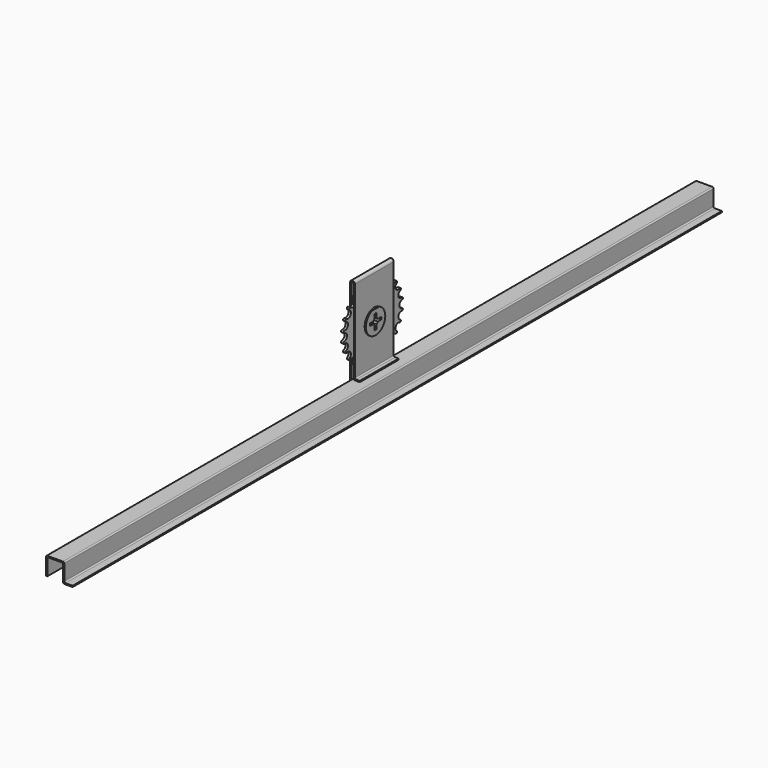
from build123d import *

# Parameters (mm, degrees)
F7_DEPTH      = 335
F1_R          = 1
F3_DEPTH      = 2
F9_DEPTH      = 2
F9_DEPTH_BACK = 4
F10_DEPTH     = 20
F11_DEPTH     = 25
F6_R          = 1


with BuildPart() as f7:
    # F0 (on Front) → F7 (new body, symmetric)
    with BuildSketch(Plane.XZ):
        Polygon((1, 0), (0, 0), (0, -1), (0, -15), (1, -15), (1, -1), (14, -1), (14, -15), (14, -16), (15, -16), (21.9038559089, -16), (21.9038559089, -15), (15, -15), (15, -1), (15, 0), (14, 0), align=None)
    extrude(amount=F7_DEPTH, both=True)

    # F1
    f1_edges = [f7.edges().sort_by_distance(p)[0] for p in [
        (15, 0, 0),
        (0, 0, 0),
        (15, 0, -15),
        (14, 0, -16),
        (14, 0, -1),
    ]]
    fillet(f1_edges, radius=F1_R)


with BuildPart() as f3:
    # F2 (on Right) → F3 (new body)
    with BuildSketch(Plane.YZ):
        with BuildLine():
            ThreePointArc((-29.8037906123, 37.9935767697), (-27, 35), (-29.8037906123, 32.0064232303))
            ThreePointArc((-29.8037906123, 32.0064232303), (-30.6596270407, 30.963583525), (-29.5630457547, 30.1777844881))
            ThreePointArc((-29.5630457547, 30.1777844881), (-26.0799973098, 28.0118857822), (-28.0134563928, 24.3946382584))
            ThreePointArc((-28.0134563928, 24.3946382584), (-28.5702241253, 23.1658256873), (-27.3076281842, 22.6906182246))
            ThreePointArc((-27.3076281842, 22.6906182246), (-23.3826859022, 21.5), (-24.3140514145, 17.5055911631))
            ThreePointArc((-24.3140514145, 17.5055911631), (-24.5338076503, 16.1745472721), (-23.1912408809, 16.0423159868))
            ThreePointArc((-23.1912408809, 16.0423159868), (-19.091883092, 15.908116908), (-18.9576840132, 11.8087591191))
            ThreePointArc((-18.9576840132, 11.8087591191), (-18.8254527279, 10.4661923497), (-17.4944088369, 10.6859485855))
            ThreePointArc((-17.4944088369, 10.6859485855), (-13.5, 11.6173140978), (-12.3093817754, 7.6923718158))
            ThreePointArc((-12.3093817754, 7.6923718158), (-11.8341743127, 6.4297758747), (-10.6053617416, 6.9865436072))
            ThreePointArc((-10.6053617416, 6.9865436072), (-6.9881142178, 8.9200026902), (-4.8222155119, 5.4369542453))
            ThreePointArc((-4.8222155119, 5.4369542453), (-4.036416475, 4.3403729593), (-2.9935767697, 5.1962093877))
            ThreePointArc((-2.9935767697, 5.1962093877), (0, 8), (2.9935767697, 5.1962093877))
            ThreePointArc((2.9935767697, 5.1962093877), (4.036416475, 4.3403729593), (4.8222155119, 5.4369542453))
            ThreePointArc((4.8222155119, 5.4369542453), (6.9881142178, 8.9200026902), (10.6053617416, 6.9865436072))
            ThreePointArc((10.6053617416, 6.9865436072), (11.8341743127, 6.4297758747), (12.3093817754, 7.6923718158))
            ThreePointArc((12.3093817754, 7.6923718158), (13.5, 11.6173140978), (17.4944088369, 10.6859485855))
            ThreePointArc((17.4944088369, 10.6859485855), (18.8254527279, 10.4661923497), (18.9576840132, 11.8087591191))
            ThreePointArc((18.9576840132, 11.8087591191), (19.091883092, 15.908116908), (23.1912408809, 16.0423159868))
            ThreePointArc((23.1912408809, 16.0423159868), (24.5338076503, 16.1745472721), (24.3140514145, 17.5055911631))
            ThreePointArc((24.3140514145, 17.5055911631), (23.3826859022, 21.5), (27.3076281842, 22.6906182246))
            ThreePointArc((27.3076281842, 22.6906182246), (28.5702241253, 23.1658256873), (28.0134563928, 24.3946382584))
            ThreePointArc((28.0134563928, 24.3946382584), (26.0799973098, 28.0118857822), (29.5630457547, 30.1777844881))
            ThreePointArc((29.5630457547, 30.1777844881), (30.6596270407, 30.963583525), (29.8037906123, 32.0064232303))
            ThreePointArc((29.8037906123, 32.0064232303), (27, 35), (29.8037906123, 37.9935767697))
            ThreePointArc((29.8037906123, 37.9935767697), (30.6596270407, 39.036416475), (29.5630457547, 39.8222155119))
            ThreePointArc((29.5630457547, 39.8222155119), (26.0799973098, 41.9881142178), (28.0134563928, 45.6053617416))
            ThreePointArc((28.0134563928, 45.6053617416), (28.5702241253, 46.8341743127), (27.3076281842, 47.3093817754))
            ThreePointArc((27.3076281842, 47.3093817754), (23.3826859022, 48.5), (24.3140514145, 52.4944088369))
            ThreePointArc((24.3140514145, 52.4944088369), (24.5338076503, 53.8254527279), (23.1912408809, 53.9576840132))
            ThreePointArc((23.1912408809, 53.9576840132), (19.091883092, 54.091883092), (18.9576840132, 58.1912408809))
            ThreePointArc((18.9576840132, 58.1912408809), (18.8254527279, 59.5338076503), (17.4944088369, 59.3140514145))
            ThreePointArc((17.4944088369, 59.3140514145), (13.5, 58.3826859022), (12.3093817754, 62.3076281842))
            ThreePointArc((12.3093817754, 62.3076281842), (11.8341743127, 63.5702241253), (10.6053617416, 63.0134563928))
            ThreePointArc((10.6053617416, 63.0134563928), (6.9881142178, 61.0799973098), (4.8222155119, 64.5630457547))
            ThreePointArc((4.8222155119, 64.5630457547), (4.036416475, 65.6596270407), (2.9935767697, 64.8037906123))
            ThreePointArc((2.9935767697, 64.8037906123), (0, 62), (-2.9935767697, 64.8037906123))
            ThreePointArc((-2.9935767697, 64.8037906123), (-4.036416475, 65.6596270407), (-4.8222155119, 64.5630457547))
            ThreePointArc((-4.8222155119, 64.5630457547), (-6.9881142178, 61.0799973098), (-10.6053617416, 63.0134563928))
            ThreePointArc((-10.6053617416, 63.0134563928), (-11.8341743127, 63.5702241253), (-12.3093817754, 62.3076281842))
            ThreePointArc((-12.3093817754, 62.3076281842), (-13.5, 58.3826859022), (-17.4944088369, 59.3140514145))
            ThreePointArc((-17.4944088369, 59.3140514145), (-18.8254527279, 59.5338076503), (-18.9576840132, 58.1912408809))
            ThreePointArc((-18.9576840132, 58.1912408809), (-19.091883092, 54.091883092), (-23.1912408809, 53.9576840132))
            ThreePointArc((-23.1912408809, 53.9576840132), (-24.5338076503, 53.8254527279), (-24.3140514145, 52.4944088369))
            ThreePointArc((-24.3140514145, 52.4944088369), (-23.3826859022, 48.5), (-27.3076281842, 47.3093817754))
            ThreePointArc((-27.3076281842, 47.3093817754), (-28.5702241253, 46.8341743127), (-28.0134563928, 45.6053617416))
            ThreePointArc((-28.0134563928, 45.6053617416), (-26.0799973098, 41.9881142178), (-29.5630457547, 39.8222155119))
            ThreePointArc((-29.5630457547, 39.8222155119), (-29.5857814733, 39.8264429327), (-29.6086158461, 39.8301001724))
            ThreePointArc((-29.6086158461, 39.8301001724), (-30.6596270407, 39.036416475), (-29.8498486408, 37.99775518))
            ThreePointArc((-29.8498486408, 37.99775518), (-29.8268457671, 37.9953778317), (-29.8037906123, 37.9935767697))
        make_face()
        with BuildLine():
            ThreePointArc((3.6960299928, 44.2918976691), (0, 25), (-3.6960299928, 44.2918976691))
            Line((-3.6960299928, 44.2918976691), (3.6960299928, 44.2918976691))
        make_face(mode=Mode.SUBTRACT)
    extrude(amount=F3_DEPTH)


with BuildPart() as f9:
    # F8 (on face) → F9 (new body, two sides)
    with BuildSketch(Plane.YZ.offset(2)) as f9_sk:
        with BuildLine():
            Line((3.6960299928, 44.2918976691), (-3.6960299928, 44.2918976691))
            ThreePointArc((-3.6960299928, 44.2918976691), (0, 25), (3.6960299928, 44.2918976691))
        make_face()
        with BuildLine():
            ThreePointArc((-2.2912878475, 36), (-1.767766953, 36.767766953), (-1, 37.2912878475))
            Line((-1, 37.2912878475), (-1, 41))
            Line((-1, 41), (1, 41))
            Line((1, 41), (1, 37.2912878475))
            ThreePointArc((1, 37.2912878475), (1.767766953, 36.767766953), (2.2912878475, 36))
            Line((2.2912878475, 36), (6, 36))
            Line((6, 36), (6, 34))
            Line((6, 34), (2.2912878475, 34))
            ThreePointArc((2.2912878475, 34), (1.767766953, 33.232233047), (1, 32.7087121525))
            Line((1, 32.7087121525), (1, 29))
            Line((1, 29), (-1, 29))
            Line((-1, 29), (-1, 32.7087121525))
            ThreePointArc((-1, 32.7087121525), (-1.767766953, 33.232233047), (-2.2912878475, 34))
            Line((-2.2912878475, 34), (-6, 34))
            Line((-6, 34), (-6, 36))
            Line((-6, 36), (-2.2912878475, 36))
        make_face(mode=Mode.SUBTRACT)
    extrude(amount=F9_DEPTH)
    extrude(f9_sk.sketch, amount=-F9_DEPTH_BACK)


with BuildPart() as f10:
    # F4 (on Front) → F10 (new body, symmetric)
    with BuildSketch(Plane.XZ):
        with BuildLine():
            Line((0, 25), (0, 44.2918976691))
            Line((0, 44.2918976691), (0, 70))
            ThreePointArc((0, 70), (1, 71), (2, 70))
            Line((2, 70), (2, 44.2918976691))
            Line((2, 44.2918976691), (2, 25))
            Line((2, 25), (2, 1))
            Line((2, 1), (2, 0))
            Line((2, 0), (3, 0))
            Line((3, 0), (7, 0))
            Line((7, 0), (7, 1))
            Line((7, 1), (3, 1))
            Line((3, 1), (3, 70))
            ThreePointArc((3, 70), (1, 72), (-1, 70))
            Line((-1, 70), (-1, -15))
            Line((-1, -15), (0, -15))
            Line((0, -15), (0, 0))
            Line((0, 0), (0, 25))
        make_face()
    extrude(amount=F10_DEPTH, both=True)

    # F5 (on face) → F11 (cut)
    with BuildSketch(Plane.YZ.offset(3)):
        with BuildLine():
            ThreePointArc((3.6960299928, 44.2918976691), (0, 45), (-3.6960299928, 44.2918976691))
            ThreePointArc((-3.6960299928, 44.2918976691), (-5.6142541834, 26.7247265928), (10, 35))
            ThreePointArc((10, 35), (8.2752734072, 40.6142541834), (3.6960299928, 44.2918976691))
        make_face()
    extrude(amount=-F11_DEPTH, mode=Mode.SUBTRACT)

    # F6
    f6_edges = [f10.edges().sort_by_distance(p)[0] for p in [
        (3, 0, 1),
        (2, 0, 0),
    ]]
    fillet(f6_edges, radius=F6_R)


solid = Compound([f7.part, f3.part, f9.part, f10.part])
